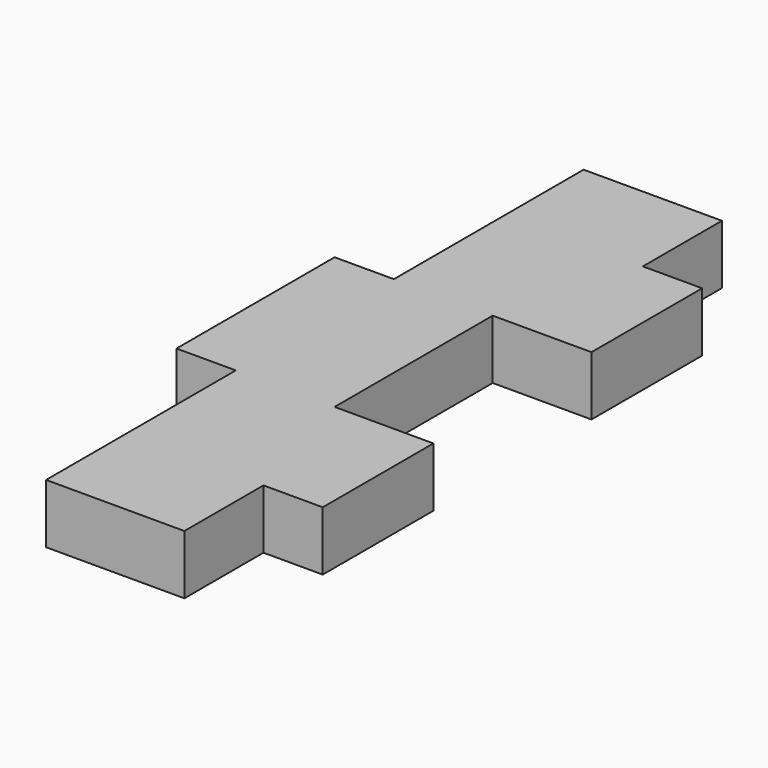
from build123d import *

# Parameters (mm, degrees)
F1_DEPTH = 3


# Not quite as in the source:
# - a feature names something its author has since deleted; it is built from what else it names


with BuildPart() as f1:
    # F0 (on Top) → F1 (new body)
    with BuildSketch(Plane.XY):
        Polygon((-8, -5), (-5, -5), (-5, -17), (2, -17), (2, -12), (5, -12), (5, -5), (0, -5), (0, 5), (5, 5), (5, 12), (2, 12), (2, 17), (-5, 17), (-5, 5), (-8, 5), align=None)
    extrude(amount=F1_DEPTH)


solid = f1.part
